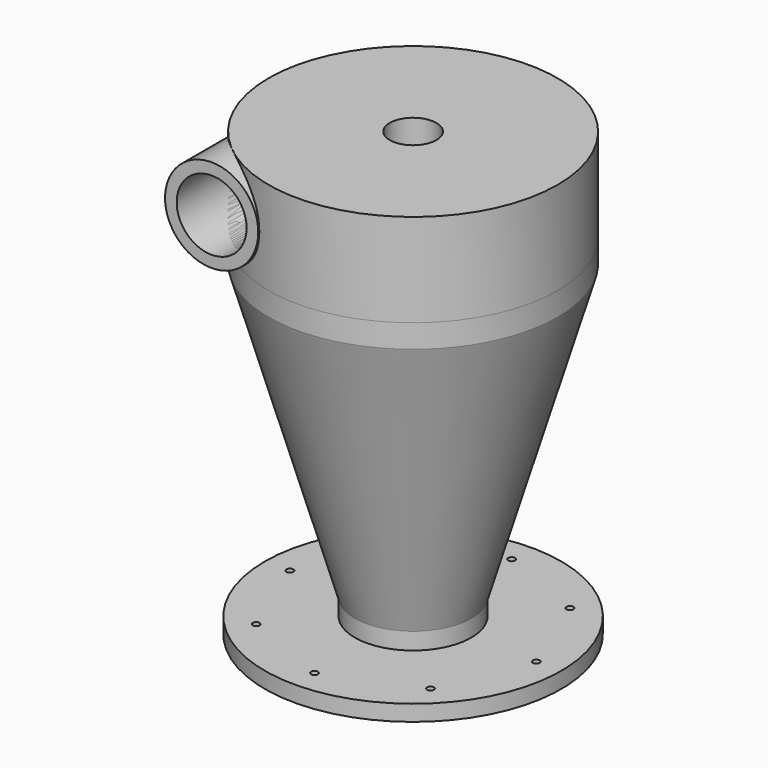
from build123d import *

# Parameters (mm, degrees)
F2_R     = 3.81
F3_DEPTH = 17.4318458885
F6_R     = 50.8
F6_R_2   = 38.1
F7_DEPTH = 151.384
F8_R     = 38.1
F9_DEPTH = 150.876


with BuildPart() as f1:
    # F0 (on Front) → F1 (revolve)
    with BuildSketch(Plane.XZ):
        Polygon((-161.5971028805, 0), (-38.1, 0), (-38.1, 17.4318458885), (-139.4343958063, 361.9006321764), (-139.4343958063, 381), (-157.5654367864, 381), (-157.5654367864, 355.6), (-63.4943762833, 35.8216682846), (-63.4943762833, 17.4318458885), (-161.5971028805, 17.4318458885), align=None)
    revolve(axis=Axis((0, 0, 239.9535179138), (0, 0, 1)))

    # F2 (on face) → F3 (cut, through all)
    with BuildSketch(Plane(origin=(0, 0, 0), x_dir=(1, 0, 0), z_dir=(0, 0, -1))):
        with Locations((95.015916754, -95.015916754)):
            Circle(F2_R)
        with Locations((0, -134.3727981148)):
            Circle(F2_R)
        with Locations((-95.015916754, -95.015916754)):
            Circle(F2_R)
        with Locations((-134.3727981148, 0)):
            Circle(F2_R)
        with Locations((-95.015916754, 95.015916754)):
            Circle(F2_R)
        with Locations((0, 134.3727981148)):
            Circle(F2_R)
        with Locations((134.3727981148, 0)):
            Circle(F2_R)
        with Locations((95.015916754, 95.015916754)):
            Circle(F2_R)
    extrude(amount=-F3_DEPTH, mode=Mode.SUBTRACT)


with BuildPart() as f5:
    # F4 (on Front) → F5 (revolve)
    with BuildSketch(Plane.XZ):
        Polygon((-139.1803958063, 381), (-139.1803958063, 368.3), (-136.6403958063, 368.3), (-136.6403958063, 469.9), (-38.795273751, 469.9), (-38.795273751, 377.8312887669), (-25.4, 377.8312887669), (-25.4, 482.6), (-38.795273751, 482.6), (-157.5654367864, 482.6), (-157.5654367864, 469.9), (-157.5654367864, 381), align=None)
    revolve(axis=Axis((0, 0, 239.9535179138), (0, 0, 1)))

    # F8 (on Front) → F9 (cut)
    with BuildSketch(Plane.XZ):
        with Locations((-98.5403958063, 431.8)):
            Circle(F8_R)
    extrude(amount=F9_DEPTH, mode=Mode.SUBTRACT)


with BuildPart() as f7:
    # F6 (on Front) → F7 (new body)
    with BuildSketch(Plane.XZ):
        with Locations((-98.5403958063, 431.8)):
            Circle(F6_R)
        with Locations((-98.5403958063, 431.8)):
            Circle(F6_R_2, mode=Mode.SUBTRACT)
    extrude(amount=F7_DEPTH)


solid = Compound([f1.part, f5.part, f7.part])
